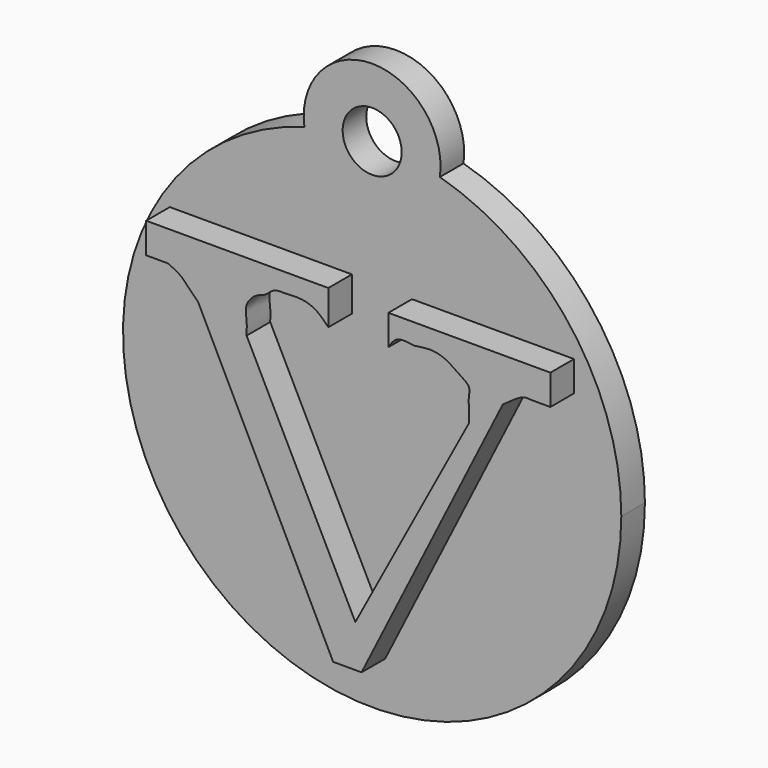
from build123d import *

# Parameters (mm, degrees)
F2_DEPTH = 4
F3_DEPTH = 8
F4_D     = 8


with BuildPart() as f2:
    # F0 (on Front) → F2 (new body)
    with BuildSketch(Plane.XZ):
        with BuildLine():
            ThreePointArc((-14.5860280627, 37.3082353296), (-25.7721388072, -22.1079707805), (28.3610324481, 4.8181205057))
            ThreePointArc((28.3610324481, 4.8181205057), (21.5239565547, 25.1881245814), (3.7817585998, 37.3082353296))
            ThreePointArc((3.7817585998, 37.3082353296), (-5.4021347314, 38.5812876852), (-14.5860280627, 37.3082353296))
        make_face()
        with BuildLine():
            ThreePointArc((-14.5860280627, 37.3082353296), (-5.4021347314, 38.5812876852), (3.7817585998, 37.3082353296))
            ThreePointArc((3.7817585998, 37.3082353296), (-5.4021347314, 47.8529951342), (-14.5860280627, 37.3082353296))
        make_face()
    extrude(amount=F2_DEPTH)

    # F1 (on Front) → F3 (join)
    with BuildSketch(Plane.XZ):
        with BuildLine():
            Line((-4.4812308624, -16.8456733227), (-19.2153304815, 12.5339938145))
            add(Edge.make_bspline(
                [(-19.2153304815, 12.5339938145), (-19.187462489, 13.0831996069), (-19.1294936303, 14.2256153377), (-19.5971693345, 16.2617964648), (-17.8782485083, 17.9666592712), (-16.6275418026, 18.0902554056), (-15.6181704414, 19.3512209953), (-13.9181197744, 19.2424127885), (-11.7824548248, 19.4327511912), (-9.7234432074, 18.78281747), (-8.6760339336, 17.6903028041), (-8.1412922591, 17.1325331371)],
                knots=[0, 0, 0, 0, 0.1071084643, 0.2227988055, 0.3430054249, 0.4340300552, 0.531806279, 0.6362553536, 0.7573294755, 0.8761076058, 1, 1, 1, 1], degree=3))
            Line((-8.1412922591, 17.1325331371), (-8.1412922591, 21.8196045607))
            Line((-8.1412922591, 21.8196045607), (-32.823253423, 21.8196045607))
            Line((-32.823253423, 21.8196045607), (-32.823253423, 17.6903028041))
            Line((-32.823253423, 17.6903028041), (-29.82012555, 17.6903028041))
            add(Edge.make_bspline(
                [(-29.82012555, 17.6903028041), (-29.2063598721, 17.3976096984), (-28.0591181767, 16.8505120895), (-27.1198992634, 15.6946853483), (-26.2472646135, 14.852226462), (-25.7846731693, 14.4056314602)],
                knots=[0, 0, 0, 0, 0.3509068735, 0.6559099195, 1, 1, 1, 1], degree=3))
            Line((-25.7846731693, 14.4056314602), (-7.4853163581, -22.570386529))
            Line((-7.4853163581, -22.570386529), (-3.6366009153, -22.570386529))
            Line((-3.6366009153, -22.570386529), (15.5083434656, 15.6256519258))
            add(Edge.make_bspline(
                [(15.5083434656, 15.6256519258), (16.0368847546, 16.0146436885), (17.0238298067, 16.7410079357), (18.3620600475, 17.5065309977), (18.870715753, 17.4367319386), (19.0745573491, 17.4087602645)],
                knots=[0, 0, 0, 0, 0.4086138264, 0.763004523, 1, 1, 1, 1], degree=3))
            Line((19.0745573491, 17.4087602645), (21.9529736787, 17.4087602645))
            Line((21.9529736787, 17.4087602645), (21.9529736787, 21.5079374611))
            Line((21.9529736787, 21.5079374611), (0, 21.5079374611))
            Line((0, 21.5079374611), (0, 17.4087602645))
            add(Edge.make_bspline(
                [(0, 17.4087602645), (0.3386937554, 17.949393323), (1.0610240671, 19.1023984773), (2.6512466921, 18.8543631276), (3.4958291799, 18.7226291746)],
                knots=[0, 0, 0, 0, 0.4688904091, 1, 1, 1, 1], degree=3))
            add(Edge.make_bspline(
                [(10.9098004177, 11.8717420846), (10.9188597305, 12.4813561639), (10.935968454, 13.6326265761), (10.8225562165, 15.0366139564), (11.2426073131, 16.3445815867), (9.2157140004, 17.5146925888), (7.9119458784, 18.5112803322), (6.2229710967, 18.9887989549), (4.9082762613, 18.9351899547), (3.9727099672, 18.7943955108), (3.4958291799, 18.7226291746)],
                knots=[0, 0, 0, 0, 0.1338160834, 0.2527147957, 0.3590610282, 0.503128831, 0.6364791552, 0.7657092985, 0.880576358, 1, 1, 1, 1], degree=3))
            Line((10.9098004177, 11.8717420846), (-4.4812308624, -16.8456733227))
        make_face()
    extrude(amount=F3_DEPTH)

    # F4 (through all)
    with Locations(Plane(origin=(0, 0, 0), x_dir=(1, 0, 0), z_dir=(0, 1, 0))):
        with Locations((-5.4021347314, -38.5812876852)):
            Hole(F4_D / 2)


solid = f2.part
